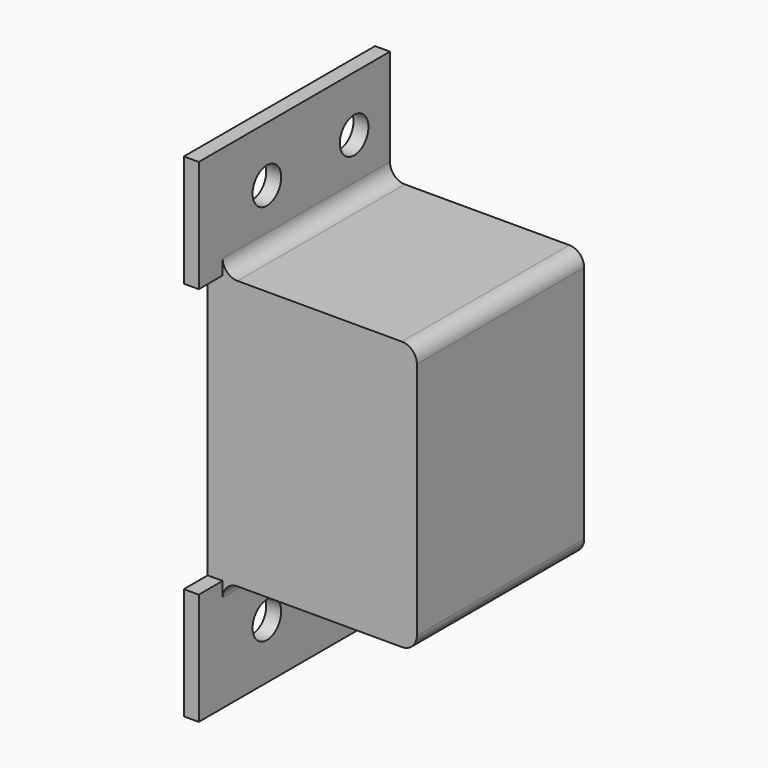
from build123d import *

# Parameters (mm, degrees)
F1_DEPTH = 25.4
F3_D     = 3.7973
F4_W     = 3.175
F4_H     = 28.575
F5_DEPTH = 22.226
F6_R     = 1.5875


with BuildPart() as f1:
    # F0 (on Front) → F1 (new body)
    with BuildSketch(Plane.XZ):
        Polygon((0, 26.19375), (0, 0), (0, -26.19375), (1.5875, -26.19375), (1.5875, -14.2875), (22.225, -14.2875), (22.225, 0), (22.225, 14.2875), (1.5875, 14.2875), (1.5875, 26.19375), align=None)
    extrude(amount=F1_DEPTH)

    # F3 (through all)
    with Locations(Plane.YZ.offset(1.5875)):
        with Locations((-16.35125, 20.32), (-4.7625, 20.32), (-16.35125, -20.32), (-4.7625, -20.32)):
            Hole(F3_D / 2)

    # F4 (on face) → F5 (cut, through all)
    with BuildSketch(Plane.YZ.offset(22.225)):
        with Locations((-23.8125, 0)):
            Rectangle(F4_W, F4_H)
    extrude(amount=-F5_DEPTH, mode=Mode.SUBTRACT)

    # F6
    f6_edges = [f1.edges().sort_by_distance(p)[0] for p in [
        (22.225, -11.1125, 14.2875),
        (22.225, -11.1125, -14.2875),
        (1.5875, -11.1125, 14.2875),
        (1.5875, -11.1125, -14.2875),
    ]]
    fillet(f6_edges, radius=F6_R)


solid = f1.part
